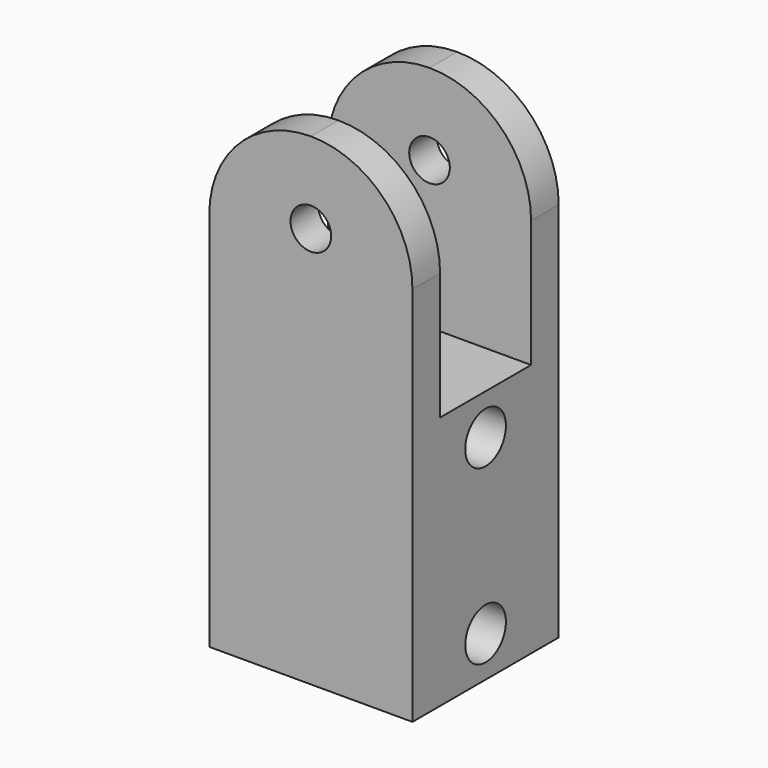
from build123d import *

# Parameters (mm, degrees)
F0_W     = 40
F0_H     = 36
F1_DEPTH = 50
F2_R     = 5
F3_DEPTH = 45
F4_W     = 40
F4_H     = 6.8
F5_DEPTH = 45
F6_R     = 19.99999
F7_R     = 4
F8_DEPTH = 50


# Not quite as in the source:
# - a fillet or chamfer is up to 0.001 mm smaller than in the source, because OpenCascade refuses the exact size


with BuildPart() as f1:
    # F0 (on Top) → F1 (new body)
    with BuildSketch(Plane.XY):
        Rectangle(F0_W, F0_H)
    extrude(amount=F1_DEPTH)

    # F2 (on face) → F3 (cut)
    with BuildSketch(Plane.YZ.offset(20)):
        with Locations((0, 42)):
            Circle(F2_R)
        with Locations((0, 8)):
            Circle(F2_R)
    extrude(amount=-F3_DEPTH, mode=Mode.SUBTRACT)

    # F4 (on face) → F5 (join)
    with BuildSketch(Plane.XY.offset(50)):
        with Locations((0, -14.6)):
            Rectangle(F4_W, F4_H)
        with Locations((0, 14.6)):
            Rectangle(F4_W, F4_H)
    extrude(amount=F5_DEPTH)

    # F6 (radius 20 in the source; OpenCascade refuses exactly that, so slightly less here)
    f6_edges = [f1.edges().sort_by_distance(p)[0] for p in [
        (20, 14.6, 95),
        (20, -14.6, 95),
        (-20, 14.6, 95),
        (-20, -14.6, 95),
    ]]
    fillet(f6_edges, radius=F6_R)

    # F7 (on face) → F8 (cut)
    with BuildSketch(Plane(origin=(0, 18, 0), x_dir=(-1, 0, 0), z_dir=(0, 1, 0))):
        with Locations((0, 79)):
            Circle(F7_R)
    extrude(amount=-F8_DEPTH, mode=Mode.SUBTRACT)


solid = f1.part
